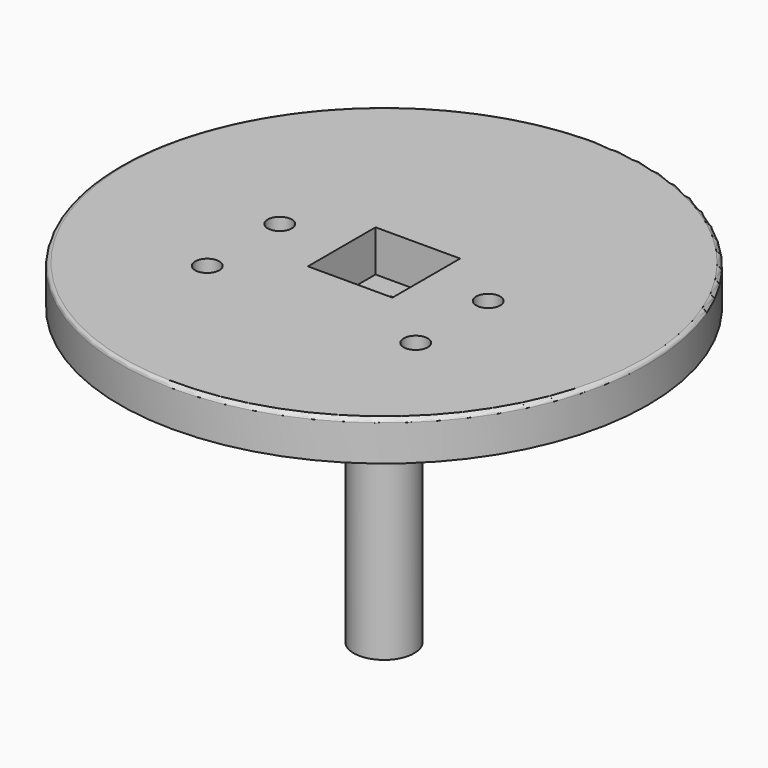
from build123d import *

# Parameters (mm, degrees)
F0_R      = 34.95
F0_R_2    = 24.925
F0_W      = 11.2
F0_H      = 11.2
F0_R_3    = 1.6
F0_R_4    = 3
F1_DEPTH  = 10
F2_R      = 0.5
F3_DEPTH  = 4.5
F4_DEPTH  = 4.75
F5_R      = 4
F5_R_2    = 1.6
F6_DEPTH  = 34.25
F7_DEPTH  = 3
F8_W      = 11.2
F8_H      = 11.2
F8_R      = 3
F8_R_2    = 1.6
F9_DEPTH  = 5.5
F10_DEPTH = 35.94117
F11_DEPTH = 8


# Not quite as in the source:
# - a feature names something its author has since deleted; it is built from what else it names


with BuildPart() as f1:
    # F0 (on Top) → F1 (new body)
    with BuildSketch(Plane.XY):
        with Locations((30.3336817496, -8.5733028001)):
            Circle(F0_R)
        with Locations((30.3336817496, -8.5733028001)):
            Circle(F0_R_2, mode=Mode.SUBTRACT)
        with Locations((30.3336817496, -8.5733028001)):
            Circle(F0_R_2)
        Polygon((18.1502625033, -17.7733028001), (19.766843257, -20.5733028001), (18.1502625033, -23.3733028001), (14.9171009958, -23.3733028001), (13.3005202421, -20.5733028001), (14.9171009958, -17.7733028001), align=None, mode=Mode.SUBTRACT)
        Polygon((45.7502625033, -17.7733028001), (47.366843257, -20.5733028001), (45.7502625033, -23.3733028001), (42.5171009958, -23.3733028001), (40.9005202421, -20.5733028001), (42.5171009958, -17.7733028001), align=None, mode=Mode.SUBTRACT)
        Polygon((42.5171009958, -11.3733028001), (40.9005202421, -8.5733028001), (42.5171009958, -5.7733028001), (45.7502625033, -5.7733028001), (47.366843257, -8.5733028001), (45.7502625033, -11.3733028001), align=None, mode=Mode.SUBTRACT)
        Polygon((14.9171009958, -11.3733028001), (13.3005202421, -8.5733028001), (14.9171009958, -5.7733028001), (18.1502625033, -5.7733028001), (19.766843257, -8.5733028001), (18.1502625033, -11.3733028001), align=None, mode=Mode.SUBTRACT)
        with Locations((30.3336817496, -8.5733028001)):
            Rectangle(F0_W, F0_H, mode=Mode.SUBTRACT)
        Polygon((42.5171009958, -5.7733028001), (40.9005202421, -8.5733028001), (42.5171009958, -11.3733028001), (45.7502625033, -11.3733028001), (47.366843257, -8.5733028001), (45.7502625033, -5.7733028001), align=None)
        with Locations((44.1336817496, -8.5733028001)):
            Circle(F0_R_3, mode=Mode.SUBTRACT)
        Polygon((45.7502625033, -23.3733028001), (47.366843257, -20.5733028001), (45.7502625033, -17.7733028001), (42.5171009958, -17.7733028001), (40.9005202421, -20.5733028001), (42.5171009958, -23.3733028001), align=None)
        with Locations((44.1336817496, -20.5733028001)):
            Circle(F0_R_3, mode=Mode.SUBTRACT)
        Polygon((18.1502625033, -23.3733028001), (19.766843257, -20.5733028001), (18.1502625033, -17.7733028001), (14.9171009958, -17.7733028001), (13.3005202421, -20.5733028001), (14.9171009958, -23.3733028001), align=None)
        with Locations((16.5336817496, -20.5733028001)):
            Circle(F0_R_3, mode=Mode.SUBTRACT)
        Polygon((14.9171009958, -5.7733028001), (13.3005202421, -8.5733028001), (14.9171009958, -11.3733028001), (18.1502625033, -11.3733028001), (19.766843257, -8.5733028001), (18.1502625033, -5.7733028001), align=None)
        with Locations((16.5336817496, -8.5733028001)):
            Circle(F0_R_3, mode=Mode.SUBTRACT)
        with Locations((30.3336817496, -8.5733028001)):
            Rectangle(F0_W, F0_H)
        with Locations((30.3336817496, -8.5733028001)):
            Circle(F0_R_4, mode=Mode.SUBTRACT)
        with Locations((30.3336817496, -8.5733028001)):
            Circle(F0_R_4)
        with Locations((30.3336817496, -8.5733028001)):
            Circle(F0_R_3, mode=Mode.SUBTRACT)
    extrude(amount=F1_DEPTH)

    # F2
    f2_edges = [f1.edges().sort_by_distance(p)[0] for p in [
        (-4.616318, -8.573303, 10),
    ]]
    fillet(f2_edges, radius=F2_R)

    # F0 (on Top) → F3 (join)
    with BuildSketch(Plane.XY):
        with Locations((30.3336817496, -8.5733028001)):
            Rectangle(F0_W, F0_H)
        with Locations((30.3336817496, -8.5733028001)):
            Circle(F0_R_4, mode=Mode.SUBTRACT)
        Polygon((18.1502625033, -23.3733028001), (19.766843257, -20.5733028001), (18.1502625033, -17.7733028001), (14.9171009958, -17.7733028001), (13.3005202421, -20.5733028001), (14.9171009958, -23.3733028001), align=None)
        with Locations((16.5336817496, -20.5733028001)):
            Circle(F0_R_3, mode=Mode.SUBTRACT)
        Polygon((45.7502625033, -23.3733028001), (47.366843257, -20.5733028001), (45.7502625033, -17.7733028001), (42.5171009958, -17.7733028001), (40.9005202421, -20.5733028001), (42.5171009958, -23.3733028001), align=None)
        with Locations((44.1336817496, -20.5733028001)):
            Circle(F0_R_3, mode=Mode.SUBTRACT)
    extrude(amount=F3_DEPTH)

    # F0 (on Top) → F4 (cut)
    with BuildSketch(Plane.XY):
        with Locations((30.3336817496, -8.5733028001)):
            Circle(F0_R)
        with Locations((30.3336817496, -8.5733028001)):
            Circle(F0_R_2, mode=Mode.SUBTRACT)
    extrude(amount=F4_DEPTH, mode=Mode.SUBTRACT)

    # F5 (on face) + F0 (on Top) → F6 (join)
    with BuildSketch(Plane(origin=(0, 0, 0), x_dir=(1, 0, 0), z_dir=(0, 0, -1))):
        with Locations((30.3336817496, 8.5733028001)):
            Circle(F5_R)
        with Locations((30.3336817496, 8.5733028001)):
            Circle(F5_R_2, mode=Mode.SUBTRACT)
    with BuildSketch(Plane.XY):
        with Locations((30.3336817496, -8.5733028001)):
            Circle(F0_R_4)
        with Locations((30.3336817496, -8.5733028001)):
            Circle(F0_R_3, mode=Mode.SUBTRACT)
    extrude(amount=F6_DEPTH, dir=(0, 0, -1))

    # F0 (on Top) → F7 (cut)
    with BuildSketch(Plane.XY):
        Polygon((45.7502625033, -23.3733028001), (47.366843257, -20.5733028001), (45.7502625033, -17.7733028001), (42.5171009958, -17.7733028001), (40.9005202421, -20.5733028001), (42.5171009958, -23.3733028001), align=None)
        with Locations((44.1336817496, -20.5733028001)):
            Circle(F0_R_3, mode=Mode.SUBTRACT)
        Polygon((42.5171009958, -5.7733028001), (40.9005202421, -8.5733028001), (42.5171009958, -11.3733028001), (45.7502625033, -11.3733028001), (47.366843257, -8.5733028001), (45.7502625033, -5.7733028001), align=None)
        with Locations((44.1336817496, -8.5733028001)):
            Circle(F0_R_3, mode=Mode.SUBTRACT)
        Polygon((14.9171009958, -5.7733028001), (13.3005202421, -8.5733028001), (14.9171009958, -11.3733028001), (18.1502625033, -11.3733028001), (19.766843257, -8.5733028001), (18.1502625033, -5.7733028001), align=None)
        with Locations((16.5336817496, -8.5733028001)):
            Circle(F0_R_3, mode=Mode.SUBTRACT)
        Polygon((18.1502625033, -23.3733028001), (19.766843257, -20.5733028001), (18.1502625033, -17.7733028001), (14.9171009958, -17.7733028001), (13.3005202421, -20.5733028001), (14.9171009958, -23.3733028001), align=None)
        with Locations((16.5336817496, -20.5733028001)):
            Circle(F0_R_3, mode=Mode.SUBTRACT)
    extrude(amount=F7_DEPTH, mode=Mode.SUBTRACT)

    # F8 (on face) → F9 (cut)
    with BuildSketch(Plane.XY.offset(10)):
        with Locations((30.3336817496, -8.5733028001)):
            Rectangle(F8_W, F8_H)
        with Locations((30.3336817496, -8.5733028001)):
            Circle(F8_R, mode=Mode.SUBTRACT)
        with Locations((30.3336817496, -8.5733028001)):
            Circle(F8_R)
        with Locations((30.3336817496, -8.5733028001)):
            Circle(F8_R_2, mode=Mode.SUBTRACT)
    extrude(amount=-F9_DEPTH, mode=Mode.SUBTRACT)

    # F0 (on Top) → F10 (cut)
    with BuildSketch(Plane.XY):
        with Locations((30.3336817496, -8.5733028001)):
            Circle(F0_R_3)
    extrude(amount=-F10_DEPTH, mode=Mode.SUBTRACT)

    # F8 (on face) → F11 (cut)
    with BuildSketch(Plane.XY.offset(10)):
        with Locations((30.3336817496, -8.5733028001)):
            Circle(F8_R)
        with Locations((30.3336817496, -8.5733028001)):
            Circle(F8_R_2, mode=Mode.SUBTRACT)
    extrude(amount=-F11_DEPTH, mode=Mode.SUBTRACT)


solid = f1.part
